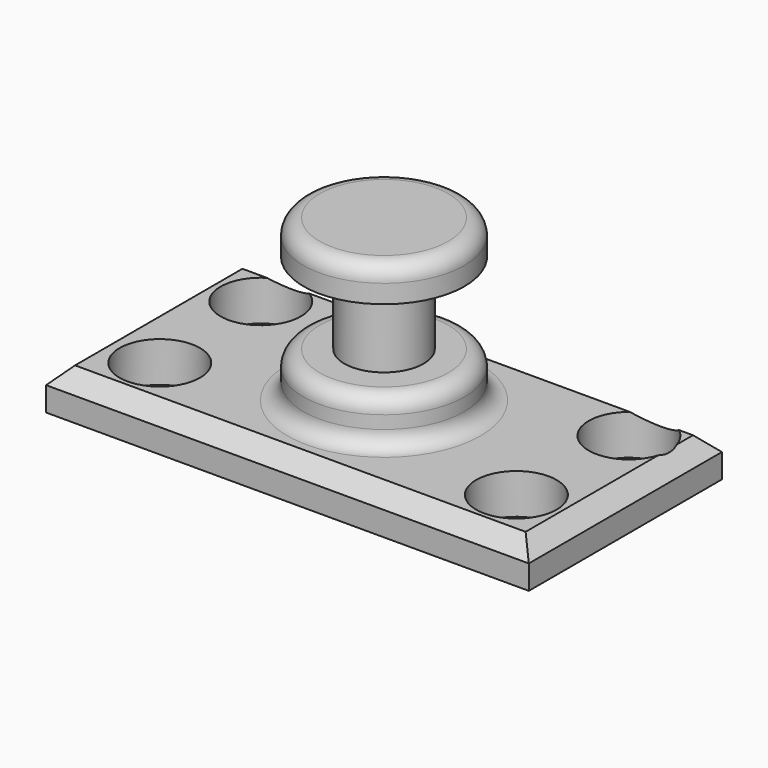
from build123d import *

# Parameters (mm, degrees)
F0_W         = 152.4
F0_H         = 76.2
F1_DEPTH     = 12.7
F2_R         = 12.7
F3_DEPTH     = 12.7
F4_R         = 12.7
F5_DEPTH     = 12.7
F6_R         = 12.7
F7_DEPTH     = 12.7
F8_W         = 25.4
F8_H         = 50.8
F11_W        = 22.735084407
F11_H        = 25.6498381495
F13_R        = 5.08
F14_T1_DEPTH = 178.5282991577
F14_T3_DEPTH = 102.3282991577


# Not quite as in the source:
# - a fillet or chamfer that OpenCascade refuses, or shapes differently, is made with other operations: its cross-section is extruded or revolved along the edge and cut away or added


with BuildPart() as f1:
    # F0 (on Top) → F1 (new body)
    with BuildSketch(Plane.XY):
        Rectangle(F0_W, F0_H)
    extrude(amount=F1_DEPTH)

    # F2 (on face) → F3 (cut)
    with BuildSketch(Plane.XY.offset(12.7)):
        with Locations((57.0033815651, -19.0182915657)):
            Circle(F2_R)
    extrude(amount=-F3_DEPTH, mode=Mode.SUBTRACT)

    # F4 (on Top) → F5 (cut)
    with BuildSketch(Plane.XY):
        with Locations((-55.634457748, -18.9344183354)):
            Circle(F4_R)
    extrude(amount=F5_DEPTH, mode=Mode.SUBTRACT)

    # F6 (on Top) → F7 (cut)
    with BuildSketch(Plane.XY):
        with Locations((-56.6692140824, 22.2065947787)):
            Circle(F6_R)
        with Locations((58.9656175097, 22.9479158466)):
            Circle(F6_R)
    extrude(amount=F7_DEPTH, mode=Mode.SUBTRACT)

    # F8 (on Front) → F9 (revolve)
    with BuildSketch(Plane.XZ):
        with Locations((12.7, 38.1)):
            Rectangle(F8_W, F8_H)
    revolve(axis=Axis((0, 0, 38.1), (0, 0, 1)))

    # F11 (on Front) → F12 (revolve, cut)
    with BuildSketch(Plane.XZ):
        with Locations((-23.9009843208, 39.7863946855)):
            Rectangle(F11_W, F11_H)
    revolve(axis=Axis((0, 0, 31.6979512572), (0, 0, 1)), mode=Mode.SUBTRACT)

    # F13
    f13_edges = [f1.edges().sort_by_distance(p)[0] for p in [
        (-25.4, 0, 63.5),
        (-25.4, 0, 26.961476),
        (-25.4, 0, 12.7),
    ]]
    fillet(f13_edges, radius=F13_R)

    # F14: chamfer of 5.08 on 4 edges, made by hand

    # F14_s2 → F14_t1 (cut)
    with BuildSketch(Plane.YZ.offset(-89.2641495789)):
        Polygon((-33.02, 12.7), (-38.1, 7.62), (-38.1, 12.7), align=None)
        Polygon((33.02, 12.7), (38.1, 7.62), (38.1, 12.7), align=None)
    extrude(amount=F14_T1_DEPTH, mode=Mode.SUBTRACT)

    # F14_s4 → F14_t3 (cut)
    with BuildSketch(Plane.XZ.offset(-51.1641495789)):
        Polygon((-71.12, 12.7), (-76.2, 7.62), (-76.2, 12.7), align=None)
        Polygon((71.12, 12.7), (76.2, 7.62), (76.2, 12.7), align=None)
    extrude(amount=F14_T3_DEPTH, mode=Mode.SUBTRACT)


solid = f1.part
